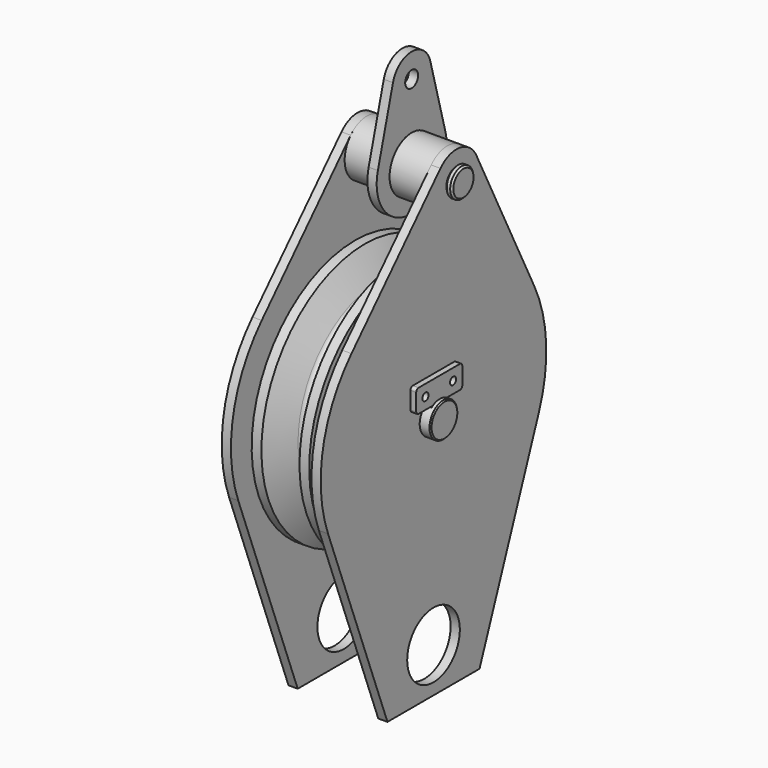
from build123d import *

# Parameters (mm, degrees)
F3_R           = 57.15
F3_R_2         = 16
F3_R_3         = 110
F3_R_4         = 45
F3_R_5         = 20
F4_DEPTH       = 16
F6_DEPTH       = 10
F7_D           = 10.8
F8_D           = 13.2
F9_R           = 30
F10_DEPTH      = 105
F11_SIZE       = 2
F12_W          = 12
F12_H          = 6
F13_DEPTH      = 50
F15_D          = 4
F15_DEPTH      = 180
F15_TIP        = 1.2017212381
F16_D          = 5.25
F16_DEPTH      = 10
F16_TIP        = 1.5772591249
F18_D          = 4.4
F18_DEPTH      = 30.001
F9_R_2         = 48
F9_R_3         = 16
F20_DEPTH      = 70
F20_DEPTH_BACK = 70
F9_R_4         = 14
F21_DEPTH      = 8
F22_R          = 15
F23_DEPTH      = 190
F22_R_2        = 25
F22_R_3        = 16
F24_DEPTH      = 12
F25_SIZE       = 3


# Not quite as in the source:
# - a pattern or mirror of a feature is missing from the dataset's text; its kind, count and spacing are read off the source's solid
# - a feature names something its author has since deleted; it is built from what else it names


with BuildPart() as f2:
    # F1 (on Front) → F2 (revolve)
    with BuildSketch(Plane.XZ):
        with BuildLine():
            Line((-70, 110), (-70, 45))
            Line((-70, 45), (-64, 45))
            Line((-64, 45), (-64, 49))
            Line((-64, 49), (-60, 49))
            Line((-60, 49), (-60, 45))
            Line((-60, 45), (-37, 45))
            Line((-37, 45), (-37, 37.5))
            Line((-37, 37.5), (37, 37.5))
            Line((37, 37.5), (37, 45))
            Line((37, 45), (60, 45))
            Line((60, 45), (60, 49))
            Line((60, 49), (64, 49))
            Line((64, 49), (64, 45))
            Line((64, 45), (70, 45))
            Line((70, 45), (70, 110))
            Line((70, 110), (60, 110))
            ThreePointArc((60, 110), (52.9289321881, 112.9289321881), (50, 120))
            Line((50, 120), (50, 225))
            Line((50, 225), (33.0739858902, 225))
            Line((33.0739858902, 225), (8.987940463, 175.6162885321))
            ThreePointArc((8.987940463, 175.6162885321), (0, 170), (-8.987940463, 175.6162885321))
            Line((-8.987940463, 175.6162885321), (-33.0739858902, 225))
            Line((-33.0739858902, 225), (-50, 225))
            Line((-50, 225), (-50, 120))
            ThreePointArc((-50, 120), (-52.9289321881, 112.9289321881), (-60, 110))
            Line((-60, 110), (-70, 110))
        make_face()
    revolve(axis=Axis((0, 0, 0), (1, 0, 0)))


with BuildPart() as f4:
    # F3 (on face) → F4 (new body)
    with BuildSketch(Plane(origin=(-70, 0, 0), x_dir=(0, -1, 0), z_dir=(-1, 0, 0))):
        with BuildLine():
            Line((-92.9152661016, 361.5006961615), (-219.0466707268, 109.7431366578))
            ThreePointArc((-219.0466707268, 109.7431366578), (-244.6822006361, 12.4748022789), (-229.072079932, -86.8963877017))
            Line((-229.072079932, -86.8963877017), (-100, -427.15))
            Line((-100, -427.15), (100, -427.15))
            Line((100, -427.15), (229.072079932, -86.8963877017))
            ThreePointArc((229.072079932, -86.8963877017), (240.2635616963, 47.9418493701), (178.1787621747, 168.1586414963))
            Line((178.1787621747, 168.1586414963), (-15.0915078188, 372.9453664972))
            ThreePointArc((-15.0915078188, 372.9453664972), (-56.9837115438, 387.4892384975), (-92.9152661016, 361.5006961615))
        make_face()
        with Locations((0, -350)):
            Circle(F3_R, mode=Mode.SUBTRACT)
        with Locations((-50, 340)):
            Circle(F3_R_2, mode=Mode.SUBTRACT)
        Circle(F3_R_3, mode=Mode.SUBTRACT)
        Circle(F3_R_3)
        Circle(F3_R_4, mode=Mode.SUBTRACT)
        Circle(F3_R_4)
        Circle(F3_R_5, mode=Mode.SUBTRACT)
    extrude(amount=F4_DEPTH)

    # F7 (through all)
    with Locations(Plane(origin=(-86, 0, 0), x_dir=(0, -1, 0), z_dir=(-1, 0, 0))):
        with Locations((-30, 45), (30, 45)):
            Hole(F7_D / 2)


with BuildPart() as f6:
    # F5 (on face) → F6 (new body)
    with BuildSketch(Plane(origin=(-86, 0, 0), x_dir=(0, -1, 0), z_dir=(-1, 0, 0))):
        with BuildLine():
            Line((45, 65), (-45, 65))
            ThreePointArc((-45, 65), (-48.5355339059, 63.5355339059), (-50, 60))
            Line((-50, 60), (-50, 30))
            ThreePointArc((-50, 30), (-48.5355339059, 26.4644660941), (-45, 25))
            Line((-45, 25), (45, 25))
            ThreePointArc((45, 25), (48.5355339059, 26.4644660941), (50, 30))
            Line((50, 30), (50, 60))
            ThreePointArc((50, 60), (48.5355339059, 63.5355339059), (45, 65))
        make_face()
    extrude(amount=F6_DEPTH)

    # F8 (through all)
    with Locations(Plane(origin=(-86, 0, 0), x_dir=(0, -1, 0), z_dir=(1, 0, 0))):
        with Locations((-30, -45), (30, -45)):
            Hole(F8_D / 2)


with BuildPart() as f10:
    # F9 (on Right) → F10 (new body, symmetric)
    with BuildSketch(Plane.YZ):
        Circle(F9_R)
    extrude(amount=F10_DEPTH, both=True)

    # F11
    f11_edges = [f10.edges().sort_by_distance(p)[0] for p in [
        (-105, -30, 0),
        (105, -30, 0),
    ]]
    chamfer(f11_edges, length=F11_SIZE)

    # F12 (on Front) → F13 (cut, symmetric)
    with BuildSketch(Plane.XZ):
        with Locations((-91, 27)):
            Rectangle(F12_W, F12_H)
    f13 = extrude(amount=F13_DEPTH, both=True, mode=Mode.SUBTRACT)

    # F13_copies: F13 across plane
    add(f13.mirror(Plane(origin=(0, 0, 0), x_dir=(0, 0, 1), z_dir=(1, 0, 0))), mode=Mode.SUBTRACT)

    # F15
    with Locations(Plane(origin=(-105, 0, 0), x_dir=(0, -1, 0), z_dir=(-1, 0, 0))):
        with Locations((0, 0)):
            Hole(F15_D / 2, depth=F15_DEPTH)
            with Locations((0, 0, -(F15_DEPTH + F15_TIP / 2))):  # 118° drill point
                Cone(0, F15_D / 2, F15_TIP, mode=Mode.SUBTRACT)

    # F16
    with Locations(Plane(origin=(-105, 0, 0), x_dir=(0, -1, 0), z_dir=(-1, 0, 0))):
        with Locations((0, 0)):
            Hole(F16_D / 2, depth=F16_DEPTH)
            with Locations((0, 0, -(F16_DEPTH + F16_TIP / 2))):  # 118° drill point
                Cone(0, F16_D / 2, F16_TIP, mode=Mode.SUBTRACT)

    # F18 (through all, one way)
    with BuildSketch(Plane(origin=(0, 0, 0), x_dir=(1, 0, 0), z_dir=(0, 0, -1))):
        with Locations((-40, 0), (40, 0)):
            Circle(F18_D / 2)
    extrude(amount=-F18_DEPTH, mode=Mode.SUBTRACT)


with BuildPart() as f19_1:
    # F19: instance of F4
    add(f4.part.mirror(Plane.YZ))


with BuildPart() as f19_2:
    # F19: instance of F6
    add(f6.part.mirror(Plane.YZ))


with BuildPart() as f20:
    # F9 (on Right) → F20 (new body, two sides)
    with BuildSketch(Plane.YZ) as f20_sk:
        with Locations((50, 340)):
            Circle(F9_R_2)
        with Locations((50, 340)):
            Circle(F9_R_3, mode=Mode.SUBTRACT)
    extrude(amount=F20_DEPTH)
    extrude(f20_sk.sketch, amount=-F20_DEPTH_BACK)

    # F9 (on Right) → F21 (join, symmetric)
    with BuildSketch(Plane.YZ):
        with BuildLine():
            Line((9.4618916962, 480.9846153846), (-23.3546721688, 359.8769230769))
            ThreePointArc((-23.3546721688, 359.8769230769), (50, 264), (123.3546721688, 359.8769230769))
            Line((123.3546721688, 359.8769230769), (90.5381083038, 480.9846153846))
            ThreePointArc((90.5381083038, 480.9846153846), (50, 512), (9.4618916962, 480.9846153846))
        make_face()
        with Locations((50, 340)):
            Circle(F9_R_2, mode=Mode.SUBTRACT)
        with Locations((50, 470)):
            Circle(F9_R_4, mode=Mode.SUBTRACT)
    extrude(amount=F21_DEPTH, both=True)


with BuildPart() as f23:
    # F22 (on face) → F23 (new body)
    with BuildSketch(Plane.YZ.offset(86)):
        with Locations((50, 340)):
            Circle(F22_R)
    extrude(amount=-F23_DEPTH)

    # F22 (on face) → F24 (join)
    with BuildSketch(Plane.YZ.offset(86)):
        with Locations((50, 340)):
            Circle(F22_R_2)
        with Locations((50, 340)):
            Circle(F22_R_3, mode=Mode.SUBTRACT)
        with Locations((50, 340)):
            Circle(F22_R_3)
        with Locations((50, 340)):
            Circle(F22_R, mode=Mode.SUBTRACT)
        with Locations((50, 340)):
            Circle(F22_R)
    extrude(amount=F24_DEPTH)

    # F25
    f25_edges = [f23.edges().sort_by_distance(p)[0] for p in [
        (98, 25, 340),
        (86, 25, 340),
        (-104, 35, 340),
    ]]
    chamfer(f25_edges, length=F25_SIZE)


solid = Compound([f2.part, f4.part, f6.part, f10.part, f19_1.part, f19_2.part, f20.part, f23.part])
